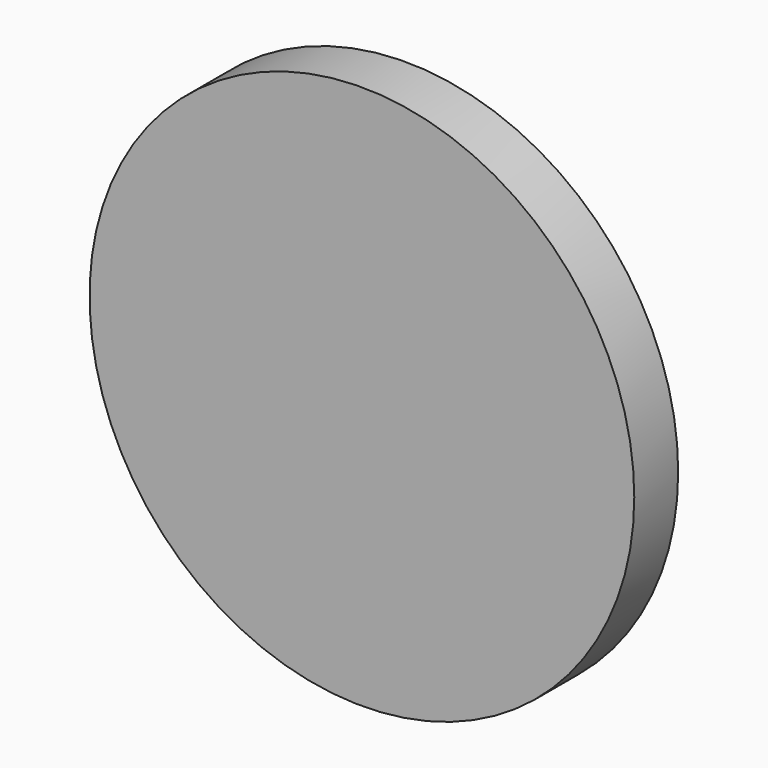
from build123d import *

# Parameters (mm, degrees)
F0_R     = 63.0399731857
F2_DEPTH = 12.7


# Not quite as in the source:
# - the program builds the solid bodies; features that only make, move or delete a surface that nothing else refers to are left out


with BuildPart() as f2:
    # F0 (on Front) → F2 (new body)
    with BuildSketch(Plane.XZ):
        Circle(F0_R)
    extrude(amount=F2_DEPTH)


solid = f2.part
